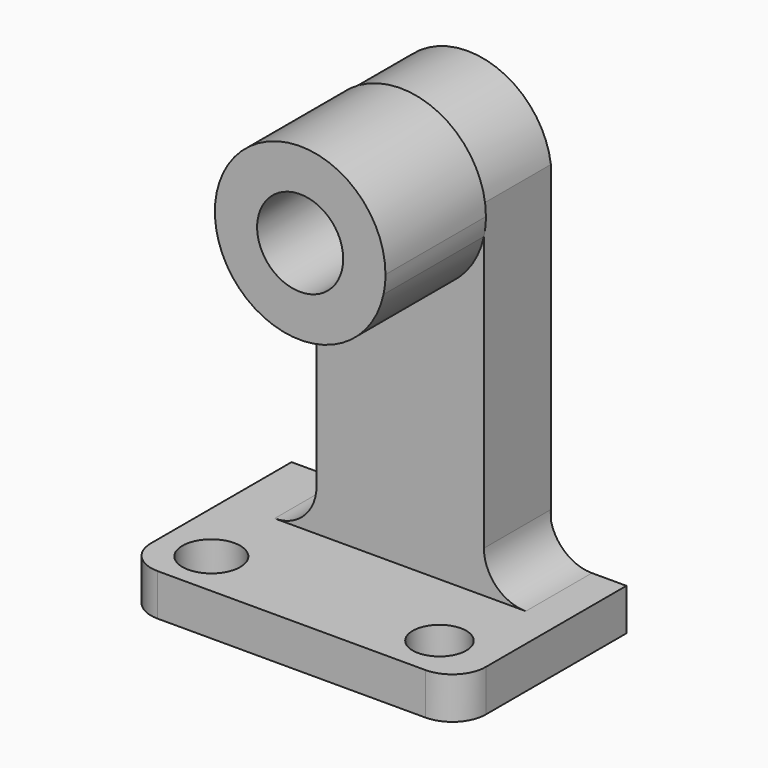
from build123d import *

# Parameters (mm, degrees)
F0_W      = 25.4
F0_H      = 69.85
F1_DEPTH  = 12.7
F3_DEPTH  = 12.701
F5_DEPTH  = 19.05
F6_R      = 6.5291939121
F7_DEPTH  = 31.751
F8_W      = 50.8
F8_H      = 31.75
F9_DEPTH  = 6.35
F10_R     = 4.3841328913
F10_R_2   = 4.0648477918
F11_DEPTH = 25.4
F13_DEPTH = 141
F14_R     = 5.08
F15_W     = 12.5349015713
F15_H     = 9.3853002578
F16_DEPTH = 12.7
F18_DEPTH = 25.4
F20_DEPTH = 12.7
F22_DEPTH = 25.4
F24_DEPTH = 25.4


# Not quite as in the source:
# - an extrude ends at something that could not be found from the text; its depth is read off the source's solid
# - a feature names something its author has since deleted; it is built from what else it names


with BuildPart() as f1:
    # F0 (on Front) → F1 (new body)
    with BuildSketch(Plane.XZ):
        with Locations((-34.1177975344, 34.925)):
            Rectangle(F0_W, F0_H)
    extrude(amount=F1_DEPTH)

    # F2 (on face) → F3 (cut, through all)
    with BuildSketch(Plane.XZ.offset(12.7)):
        with BuildLine():
            ThreePointArc((-46.8177975344, 57.1627020836), (-34.8779343498, 69.8199859011), (-21.4177975344, 58.7931149299))
            Line((-21.4177975344, 58.7931149299), (-21.4177975344, 69.85))
            Line((-21.4177975344, 69.85), (-46.8177975344, 69.85))
            Line((-46.8177975344, 69.85), (-46.8177975344, 57.1627020836))
        make_face()
    extrude(amount=-F3_DEPTH, mode=Mode.SUBTRACT)

    # F4 (on face) → F5 (join)
    with BuildSketch(Plane.XZ.offset(12.7)):
        with BuildLine():
            Line((-46.8177975344, 57.1627020836), (-46.8177975344, 54.9187152869))
            ThreePointArc((-46.8177975344, 54.9187152869), (-34.3603071914, 44.1520357407), (-21.4177975344, 54.3305374906))
            Line((-21.4177975344, 54.3305374906), (-21.4177975344, 58.7931149299))
            ThreePointArc((-21.4177975344, 58.7931149299), (-34.8779343498, 69.8199859011), (-46.8177975344, 57.1627020836))
        make_face()
        with BuildLine():
            ThreePointArc((-21.4177975344, 54.3305374906), (-21.194958074, 55.7017298658), (-21.1203918045, 57.0889089552))
            ThreePointArc((-21.1203918045, 57.0889089552), (-35.1496925912, 69.9833496353), (-46.8177975344, 54.9187152869))
            Line((-46.8177975344, 54.9187152869), (-46.8177975344, 57.1627020836))
            ThreePointArc((-46.8177975344, 57.1627020836), (-34.8779343498, 69.8199859011), (-21.4177975344, 58.7931149299))
            Line((-21.4177975344, 58.7931149299), (-21.4177975344, 54.3305374906))
        make_face()
    extrude(amount=F5_DEPTH)

    # F6 (on face) → F7 (cut, through all)
    with BuildSketch(Plane.XZ.offset(31.75)):
        with Locations((-34.0607331136, 57.0889089552)):
            Circle(F6_R)
    extrude(amount=-F7_DEPTH, mode=Mode.SUBTRACT)

    # F8 (on Top) → F9 (join)
    with BuildSketch(Plane.XY):
        with Locations((-35.2321754485, -16.0400984287)):
            Rectangle(F8_W, F8_H)
    extrude(amount=F9_DEPTH)

    # F10 (on face) → F11 (cut)
    with BuildSketch(Plane.XY.offset(6.35)):
        with Locations((-52.9474318027, -24.9871537089)):
            Circle(F10_R)
        with Locations((-18.3323584497, -24.9871537089)):
            Circle(F10_R_2)
    extrude(amount=-F11_DEPTH, mode=Mode.SUBTRACT)

    # F12 (on Front) → F13 (cut, through all)
    with BuildSketch(Plane.XZ):
        with BuildLine():
            ThreePointArc((-47.1297007382, 13.1953000858), (-48.9895726777, 17.6854281464), (-53.4797007382, 19.5453000858))
            ThreePointArc((-53.4797007382, 19.5453000858), (-57.9698287987, 17.6854281464), (-59.8297007382, 13.1953000858))
            ThreePointArc((-59.8297007382, 13.1953000858), (-57.9698287987, 8.7051720253), (-53.4797007382, 6.8453000858))
            ThreePointArc((-53.4797007382, 6.8453000858), (-48.9895726777, 8.7051720253), (-47.1297007382, 13.1953000858))
        make_face()
        with BuildLine():
            ThreePointArc((-59.8297007382, 13.1953000858), (-57.9698287987, 17.6854281464), (-53.4797007382, 19.5453000858))
            Line((-53.4797007382, 19.5453000858), (-59.8297007382, 19.5453000858))
            Line((-59.8297007382, 19.5453000858), (-59.8297007382, 13.1953000858))
        make_face()
        with BuildLine():
            ThreePointArc((-53.4797007382, 6.8453000858), (-57.9698287987, 8.7051720253), (-59.8297007382, 13.1953000858))
            Line((-59.8297007382, 13.1953000858), (-59.8297007382, 6.8453000858))
            Line((-59.8297007382, 6.8453000858), (-53.4797007382, 6.8453000858))
        make_face()
        with BuildLine():
            Line((-47.1297007382, 13.1953000858), (-47.1297007382, 19.5453000858))
            Line((-47.1297007382, 19.5453000858), (-53.4797007382, 19.5453000858))
            ThreePointArc((-53.4797007382, 19.5453000858), (-48.9895726777, 17.6854281464), (-47.1297007382, 13.1953000858))
        make_face()
        with BuildLine():
            ThreePointArc((-8.7253203213, 12.5349001028), (-14.8973108068, 18.7068905883), (-21.0693012923, 12.5349001028))
            ThreePointArc((-21.0693012923, 12.5349001028), (-19.2615671325, 8.170643777), (-14.8973108068, 6.3629096172))
            ThreePointArc((-14.8973108068, 6.3629096172), (-10.533054481, 8.170643777), (-8.7253203213, 12.5349001028))
        make_face()
    extrude(amount=-F13_DEPTH, mode=Mode.SUBTRACT)

    # F14
    f14_edges = [f1.edges().sort_by_distance(p)[0] for p in [
        (-9.832175, -31.915098, 3.175),
        (-60.632175, -31.915098, 3.175),
    ]]
    fillet(f14_edges, radius=F14_R)

    # F15 (on face) → F16 (join)
    with BuildSketch(Plane.YZ.offset(-21.4177975344)):
        with Locations((-6.4325492144, 11.0426501289)):
            Rectangle(F15_W, F15_H)
    extrude(amount=F16_DEPTH)

    # F17 (on face) → F18 (cut)
    with BuildSketch(Plane.XZ.offset(12.7)):
        with BuildLine():
            ThreePointArc((-20.6453823473, 15.7353002578), (-21.221664756, 14.2660198655), (-21.4177975344, 12.7))
            ThreePointArc((-21.4177975344, 12.7), (-19.5579255949, 8.2098719395), (-15.0677975344, 6.35))
            ThreePointArc((-15.0677975344, 6.35), (-10.5776694739, 8.2098719395), (-8.7177975344, 12.7))
            ThreePointArc((-8.7177975344, 12.7), (-8.9139303128, 14.2660198655), (-9.4902127215, 15.7353002578))
            Line((-9.4902127215, 15.7353002578), (-20.6453823473, 15.7353002578))
        make_face()
        with BuildLine():
            ThreePointArc((-9.4902127215, 15.7353002578), (-15.0677975344, 19.05), (-20.6453823473, 15.7353002578))
            Line((-20.6453823473, 15.7353002578), (-9.4902127215, 15.7353002578))
        make_face()
        with BuildLine():
            ThreePointArc((-8.7177975344, 12.7), (-10.5776694739, 8.2098719395), (-15.0677975344, 6.35))
            Line((-15.0677975344, 6.35), (-9.8321754485, 6.35))
            Line((-9.8321754485, 6.35), (-8.7177975344, 6.35))
            Line((-8.7177975344, 6.35), (-8.7177975344, 12.7))
        make_face()
        with BuildLine():
            Line((-8.7177975344, 15.7353002578), (-9.4902127215, 15.7353002578))
            ThreePointArc((-9.4902127215, 15.7353002578), (-8.9139303128, 14.2660198655), (-8.7177975344, 12.7))
            Line((-8.7177975344, 12.7), (-8.7177975344, 15.7353002578))
        make_face()
    extrude(amount=-F18_DEPTH, mode=Mode.SUBTRACT)

    # F19 (on face) → F20 (join)
    with BuildSketch(Plane(origin=(-46.8177975344, 0, 0), x_dir=(0, -1, 0), z_dir=(-1, 0, 0))):
        Polygon((12.7, 16.4465010166), (0, 16.4465010166), (0, 6.35), (0.1650984287, 6.35), (12.7, 6.35), align=None)
    extrude(amount=F20_DEPTH)

    # F21 (on face) → F22 (cut)
    with BuildSketch(Plane.XZ.offset(12.7)):
        with BuildLine():
            Line((-59.5177975344, 6.35), (-53.1677975344, 6.35))
            ThreePointArc((-53.1677975344, 6.35), (-57.6579255949, 8.2098719395), (-59.5177975344, 12.7))
            Line((-59.5177975344, 12.7), (-59.5177975344, 6.35))
        make_face()
        with BuildLine():
            Line((-21.4177975344, 15.7353002578), (-21.4177975344, 12.7))
            ThreePointArc((-21.4177975344, 12.7), (-21.221664756, 14.2660198655), (-20.6453823473, 15.7353002578))
            Line((-20.6453823473, 15.7353002578), (-21.4177975344, 15.7353002578))
        make_face()
        with BuildLine():
            ThreePointArc((-59.5177975344, 12.7), (-59.204311952, 14.6705313207), (-58.2948073971, 16.4465010166))
            Line((-58.2948073971, 16.4465010166), (-59.5177975344, 16.4465010166))
            Line((-59.5177975344, 16.4465010166), (-59.5177975344, 12.7))
        make_face()
        with BuildLine():
            Line((-58.2948073971, 16.4465010166), (-48.0407876717, 16.4465010166))
            ThreePointArc((-48.0407876717, 16.4465010166), (-53.1677975344, 19.05), (-58.2948073971, 16.4465010166))
        make_face()
        with BuildLine():
            ThreePointArc((-53.1677975344, 6.35), (-48.6776694739, 8.2098719395), (-46.8177975344, 12.7))
            ThreePointArc((-46.8177975344, 12.7), (-47.1312831168, 14.6705313207), (-48.0407876717, 16.4465010166))
            Line((-48.0407876717, 16.4465010166), (-58.2948073971, 16.4465010166))
            ThreePointArc((-58.2948073971, 16.4465010166), (-59.204311952, 14.6705313207), (-59.5177975344, 12.7))
            ThreePointArc((-59.5177975344, 12.7), (-57.6579255949, 8.2098719395), (-53.1677975344, 6.35))
        make_face()
    extrude(amount=-F22_DEPTH, mode=Mode.SUBTRACT)

    # F23 (on face) → F24 (cut)
    with BuildSketch(Plane.XZ.offset(12.7)):
        with BuildLine():
            Line((-46.8177975344, 12.7), (-46.8177975344, 16.4465010166))
            Line((-46.8177975344, 16.4465010166), (-48.0407876717, 16.4465010166))
            ThreePointArc((-48.0407876717, 16.4465010166), (-47.1312831168, 14.6705313207), (-46.8177975344, 12.7))
        make_face()
    extrude(amount=-F24_DEPTH, mode=Mode.SUBTRACT)


solid = f1.part
